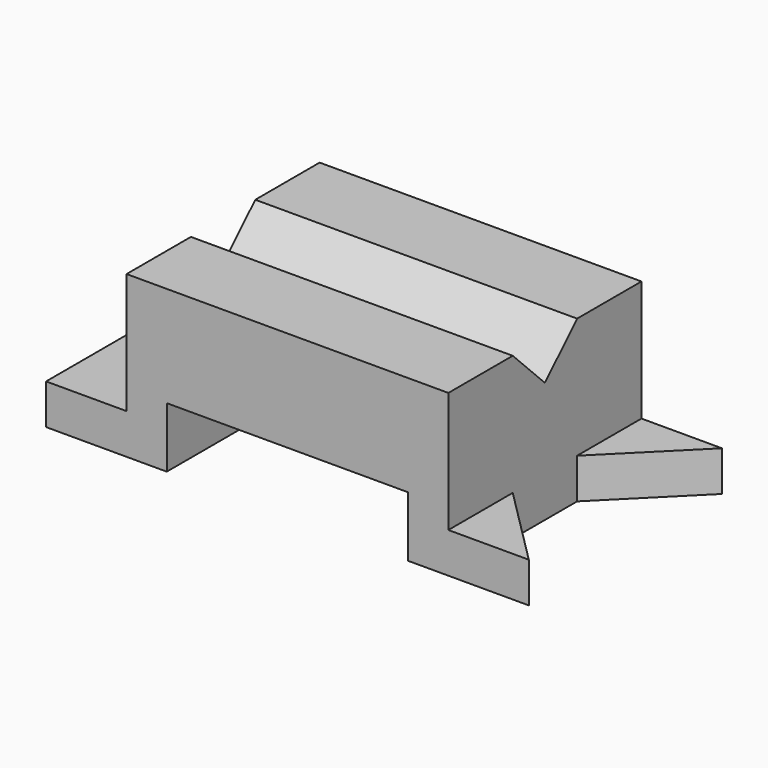
from build123d import *

# Parameters (mm, degrees)
F1_DEPTH = 50.8
F0_W     = 25.4
F0_H     = 76.2
F2_DEPTH = 12.7
F3_DEPTH = 12.7
F5_DEPTH = 25.4
F6_DEPTH = 127
F7_W     = 76.2
F7_H     = 19.05
F8_DEPTH = 101.6


with BuildPart() as f1:
    # F0 (on Top) → F1 (new body)
    with BuildSketch(Plane.XY):
        Polygon((72.5681655884, 42.7888188445), (-29.0318344116, 42.7888188445), (-29.0318344116, -33.4111811555), (72.5681655884, -33.4111811555), (72.5681655884, -8.0111811555), (72.5681655884, 17.3888188445), align=None)
    extrude(amount=F1_DEPTH)

    # F0 (on Top) → F2 (join)
    with BuildSketch(Plane.XY):
        with Locations((-41.7318344116, 4.6888188445)):
            Rectangle(F0_W, F0_H)
    extrude(amount=F2_DEPTH)

    # F0 (on Top) → F3 (join)
    with BuildSketch(Plane.XY):
        Polygon((97.9681655884, 42.7888188445), (72.5681655884, 42.7888188445), (72.5681655884, 17.3888188445), align=None)
        Polygon((72.5681655884, -8.0111811555), (72.5681655884, -33.4111811555), (97.9681655884, -33.4111811555), align=None)
    extrude(amount=F3_DEPTH)

    # F4 (on face) → F5 (join)
    with BuildSketch(Plane.YZ.offset(72.5681655884)):
        Polygon((-8.0111859904, 50.8), (4.6888188445, 38.1), (17.3888188445, 50.8), align=None)
    extrude(amount=F5_DEPTH)

    # F6 (cut): a face of the model
    f6_faces = [f1.faces().sort_by_distance(p)[0] for p in [
        (97.9681655884, 4.6888172329, 46.5666666667),
    ]]
    extrude(f6_faces, amount=-F6_DEPTH, mode=Mode.SUBTRACT)

    # F7 (on face) → F8 (cut)
    with BuildSketch(Plane.XZ.offset(33.4111811555)):
        with Locations((21.7681655884, 9.525)):
            Rectangle(F7_W, F7_H)
    extrude(amount=-F8_DEPTH, mode=Mode.SUBTRACT)


solid = f1.part
